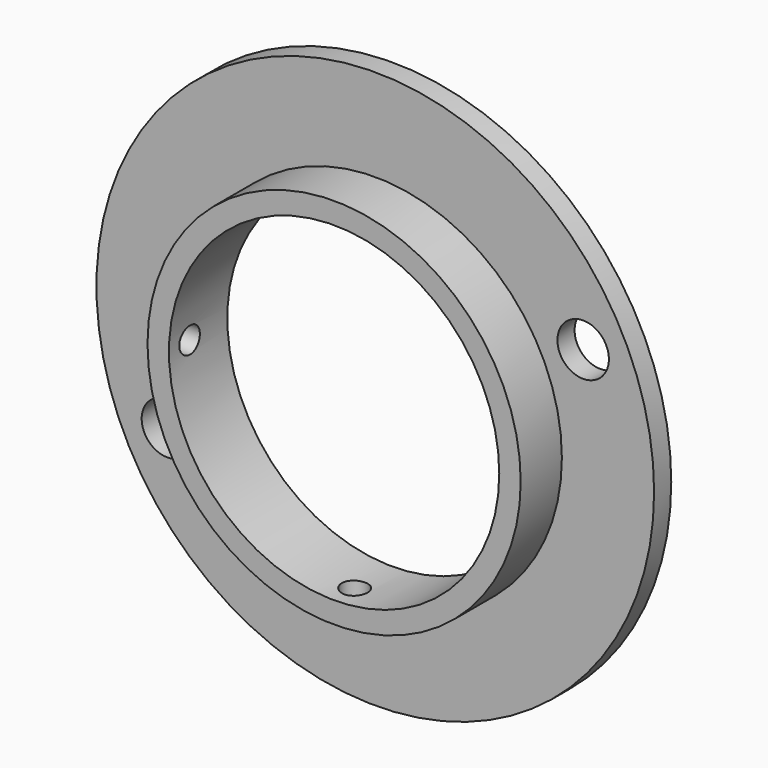
from build123d import *

# Parameters (mm, degrees)
F0_R            = 21.75
F0_R_2          = 19.25
F1_DEPTH        = 6
F2_R            = 32.5
F3_DEPTH        = 2.5
F4_R            = 19.25
F5_DEPTH        = 25
F6_R            = 1.5
F7_DEPTH        = 25
F7_COPIES_COUNT = 2
F7_COPIES_ANGLE = 90
F8_R            = 3
F9_DEPTH        = 25


# Not quite as in the source:
# - a pattern or mirror of a feature is missing from the dataset's text; its kind, count and spacing are read off the source's solid


with BuildPart() as f1:
    # F0 (on Front) → F1 (new body)
    with BuildSketch(Plane.XZ):
        Circle(F0_R)
        Circle(F0_R_2, mode=Mode.SUBTRACT)
    extrude(amount=F1_DEPTH)

    # F2 (on Front) → F3 (join)
    with BuildSketch(Plane.XZ):
        Circle(F2_R)
    extrude(amount=-F3_DEPTH)

    # F4 (on Front) → F5 (cut)
    with BuildSketch(Plane.XZ):
        Circle(F4_R)
    extrude(amount=-F5_DEPTH, mode=Mode.SUBTRACT)

    # F6 (on Top) → F7 (cut)
    with BuildSketch(Plane.XY):
        with Locations((0, -3)):
            Circle(F6_R)
    f7 = extrude(amount=-F7_DEPTH, mode=Mode.SUBTRACT)

    # F7_copies: F7 ×2 about axis
    f7_copies_axis = Axis((0, 0, 0), (0, 1, 0))
    for i in range(1, F7_COPIES_COUNT):
        add(f7.rotate(f7_copies_axis, i * F7_COPIES_ANGLE / (F7_COPIES_COUNT - 1)), mode=Mode.SUBTRACT)

    # F8 (on face) → F9 (cut)
    with BuildSketch(Plane.XZ):
        with Locations((24.2303724922, 11.9117189728)):
            Circle(F8_R)
    f9 = extrude(amount=-F9_DEPTH, mode=Mode.SUBTRACT)

    # F9_copies: F9 across plane
    add(f9.mirror(Plane(origin=(0, 0, 0), x_dir=(0.4411747768, 0, -0.8974212034), z_dir=(-0.8974212034, 0, -0.4411747768))), mode=Mode.SUBTRACT)


solid = f1.part
